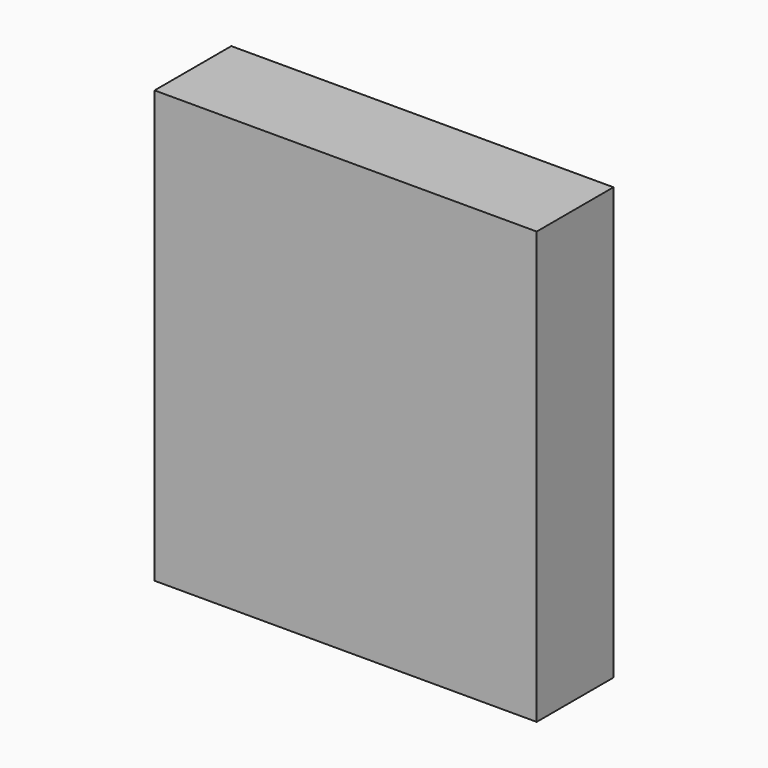
from build123d import *

# Parameters (mm, degrees)
F1_DEPTH  = 35
F2_DEPTH  = 35
F3_R      = 35
F4_DEPTH  = 99
F5_R      = 10
F6_R      = 10
F7_R      = 40
F9_DEPTH  = 23
F10_R     = 22.99999
F12_W     = 478
F12_H     = 540
F13_DEPTH = 120


# Not quite as in the source:
# - a fillet or chamfer is up to 0.001 mm smaller than in the source, because OpenCascade refuses the exact size
# - a feature names something its author has since deleted; it is built from what else it names


with BuildPart() as f1:
    # F0 (on Front) → F1 (new body)
    with BuildSketch(Plane.XZ):
        with BuildLine():
            Line((-40.7399735484, 161), (209, 161))
            ThreePointArc((209, 161), (157.3555894158, 298.5507850927), (27.9452777071, 368.1233001231))
            add(Edge.make_bspline(
                [(27.9452777071, 368.1233001231), (-41.6365018393, 325.152564643), (-43.0879443269, 262.4678679339), (-40.7399735484, 161)],
                knots=[0, 0, 0, 0, 225.5050238403, 225.5050238403, 225.5050238403, 225.5050238403], degree=3))
        make_face()
        with BuildLine():
            Line((0, -110), (209, -110))
            Line((209, -110), (209, 161))
            Line((209, 161), (-40.7399735484, 161))
            add(Edge.make_bspline(
                [(-40.7399735484, 161), (-40.5096354565, 151.0459088739), (-40.2427326078, 140.718576638), (-40, 130)],
                knots=[225.5050238403, 225.5050238403, 225.5050238403, 225.5050238403, 247.627273991, 247.627273991, 247.627273991, 247.627273991], degree=3))
            Line((-40, 130), (0, 130))
            Line((0, 130), (0, -110))
        make_face()
    extrude(amount=F1_DEPTH)

    # F5
    f5_edges = [f1.edges().sort_by_distance(p)[0] for p in [
        (-40, -17.5, 130),
    ]]
    fillet(f5_edges, radius=F5_R)

    # F6
    f6_edges = [f1.edges().sort_by_distance(p)[0] for p in [
        (0, -17.5, 130),
    ]]
    fillet(f6_edges, radius=F6_R)

    # F7
    f7_edges = [f1.edges().sort_by_distance(p)[0] for p in [
        (27.945278, -17.5, 368.1233),
    ]]
    fillet(f7_edges, radius=F7_R)

    # F8 (on face) → F9 (join)
    with BuildSketch(Plane.XZ.offset(35)):
        with BuildLine():
            Line((40, 283), (40, 237))
            ThreePointArc((40, 237), (63, 260), (40, 283))
        make_face()
        with BuildLine():
            ThreePointArc((40, 233), (17, 210), (40, 187))
            Line((40, 187), (40, 210))
            Line((40, 210), (40, 233))
        make_face()
        with BuildLine():
            ThreePointArc((40, 137), (63, 160), (40, 183))
            Line((40, 183), (40, 137))
        make_face()
        with BuildLine():
            Line((40, 87), (40, 133))
            ThreePointArc((40, 133), (17, 110), (40, 87))
        make_face()
        with BuildLine():
            ThreePointArc((40, 37), (63, 60), (40, 83))
            Line((40, 83), (40, 37))
        make_face()
        with BuildLine():
            Line((40, -13), (40, 33))
            ThreePointArc((40, 33), (17, 10), (40, -13))
        make_face()
        with BuildLine():
            Line((104.5515164733, 283.0000003353), (104.5515164733, 237.0000003353))
            ThreePointArc((104.5515164733, 237.0000003353), (127.5515164733, 260.0000003353), (104.5515164733, 283.0000003353))
        make_face()
        with BuildLine():
            ThreePointArc((104.5515164733, 233.0000003353), (81.5515164733, 210.0000003353), (104.5515164733, 187.0000003353))
            Line((104.5515164733, 187.0000003353), (104.5515164733, 210.0000003353))
            Line((104.5515164733, 210.0000003353), (104.5515164733, 233.0000003353))
        make_face()
        with BuildLine():
            ThreePointArc((104.5515164733, 137.0000003353), (127.5515164733, 160.0000003353), (104.5515164733, 183.0000003353))
            Line((104.5515164733, 183.0000003353), (104.5515164733, 137.0000003353))
        make_face()
        with BuildLine():
            Line((104.5515164733, 87.0000003353), (104.5515164733, 133.0000003353))
            ThreePointArc((104.5515164733, 133.0000003353), (81.5515164733, 110.0000003353), (104.5515164733, 87.0000003353))
        make_face()
        with BuildLine():
            ThreePointArc((104.5515164733, 37.0000003353), (127.5515164733, 60.0000003353), (104.5515164733, 83.0000003353))
            Line((104.5515164733, 83.0000003353), (104.5515164733, 37.0000003353))
        make_face()
        with BuildLine():
            Line((104.5515164733, -12.9999996647), (104.5515164733, 33.0000003353))
            ThreePointArc((104.5515164733, 33.0000003353), (81.5515164733, 10.0000003353), (104.5515164733, -12.9999996647))
        make_face()
        with BuildLine():
            ThreePointArc((165.5515581369, 232.9999997765), (142.5515581369, 209.9999997765), (165.5515581369, 186.9999997765))
            Line((165.5515581369, 186.9999997765), (165.5515581369, 209.9999997765))
            Line((165.5515581369, 209.9999997765), (165.5515581369, 232.9999997765))
        make_face()
        with BuildLine():
            Line((165.5515581369, 182.9999997765), (165.5515581369, 136.9999997765))
            ThreePointArc((165.5515581369, 136.9999997765), (188.5515581369, 159.9999997765), (165.5515581369, 182.9999997765))
        make_face()
        with BuildLine():
            Line((165.5515581369, 86.9999997765), (165.5515581369, 132.9999997765))
            ThreePointArc((165.5515581369, 132.9999997765), (142.5515581369, 109.9999997765), (165.5515581369, 86.9999997765))
        make_face()
        with BuildLine():
            ThreePointArc((165.5515581369, 36.9999997765), (188.5515581369, 59.9999997765), (165.5515581369, 82.9999997765))
            Line((165.5515581369, 82.9999997765), (165.5515581369, 36.9999997765))
        make_face()
        with BuildLine():
            Line((165.5515581369, -13.0000002235), (165.5515581369, 32.9999997765))
            ThreePointArc((165.5515581369, 32.9999997765), (142.5515581369, 9.9999997765), (165.5515581369, -13.0000002235))
        make_face()
    extrude(amount=F9_DEPTH)

    # F10 (radius 23 in the source; OpenCascade refuses exactly that, so slightly less here)
    f10_edges = [f1.edges().sort_by_distance(p)[0] for p in [
        (63, -58, 260),
        (17, -58, 210),
        (63, -58, 160),
        (17, -58, 110),
        (63, -58, 60),
        (17, -58, 10),
        (81.551516, -58, 10),
        (127.551516, -58, 60),
        (81.551516, -58, 110),
        (127.551516, -58, 160),
        (81.551516, -58, 210),
        (127.551516, -58, 260),
        (142.551558, -58, 210),
        (188.551558, -58, 160),
        (142.551558, -58, 110),
        (188.551558, -58, 60),
        (142.551558, -58, 10),
    ]]
    fillet(f10_edges, radius=F10_R)


with BuildPart() as f2:
    # F0 (on Front) → F2 (new body)
    with BuildSketch(Plane.XZ):
        with BuildLine():
            Line((-209, 161), (-40.7399735484, 161))
            add(Edge.make_bspline(
                [(27.9452777071, 368.1233001231), (-41.6365018393, 325.152564643), (-43.0879443269, 262.4678679339), (-40.7399735484, 161)],
                knots=[0, 0, 0, 0, 225.5050238403, 225.5050238403, 225.5050238403, 225.5050238403], degree=3))
            ThreePointArc((27.9452777071, 368.1233001231), (-137.5507850927, 318.3555894158), (-209, 161))
        make_face()
        with BuildLine():
            Line((-209, -110), (0, -110))
            Line((0, -110), (0, 130))
            Line((0, 130), (-40, 130))
            add(Edge.make_bspline(
                [(-40.7399735484, 161), (-40.5096354565, 151.0459088739), (-40.2427326078, 140.718576638), (-40, 130)],
                knots=[225.5050238403, 225.5050238403, 225.5050238403, 225.5050238403, 247.627273991, 247.627273991, 247.627273991, 247.627273991], degree=3))
            Line((-40.7399735484, 161), (-209, 161))
            Line((-209, 161), (-209, -110))
        make_face()
        with BuildLine():
            Line((-40.7399735484, 161), (209, 161))
            ThreePointArc((209, 161), (157.3555894158, 298.5507850927), (27.9452777071, 368.1233001231))
            add(Edge.make_bspline(
                [(27.9452777071, 368.1233001231), (-41.6365018393, 325.152564643), (-43.0879443269, 262.4678679339), (-40.7399735484, 161)],
                knots=[0, 0, 0, 0, 225.5050238403, 225.5050238403, 225.5050238403, 225.5050238403], degree=3))
        make_face()
        with BuildLine():
            Line((0, -110), (209, -110))
            Line((209, -110), (209, 161))
            Line((209, 161), (-40.7399735484, 161))
            add(Edge.make_bspline(
                [(-40.7399735484, 161), (-40.5096354565, 151.0459088739), (-40.2427326078, 140.718576638), (-40, 130)],
                knots=[225.5050238403, 225.5050238403, 225.5050238403, 225.5050238403, 247.627273991, 247.627273991, 247.627273991, 247.627273991], degree=3))
            Line((-40, 130), (0, 130))
            Line((0, 130), (0, -110))
        make_face()
    extrude(amount=-F2_DEPTH)

    # F3 (on Front) → F4 (cut)
    with BuildSketch(Plane.XZ):
        with Locations((-120, 200)):
            Circle(F3_R)
    extrude(amount=-F4_DEPTH, mode=Mode.SUBTRACT)

    # F11: union F1
    add(f1.part)


with BuildPart() as f13:
    # F12 (on face) → F13 (new body)
    with BuildSketch(Plane(origin=(0, 35, 0), x_dir=(-1, 0, 0), z_dir=(0, 1, 0))):
        with Locations((0, 130)):
            Rectangle(F12_W, F12_H)
    extrude(amount=-F13_DEPTH)

    # F14: cut F2
    add(f2.part, mode=Mode.SUBTRACT)


solid = f13.part
